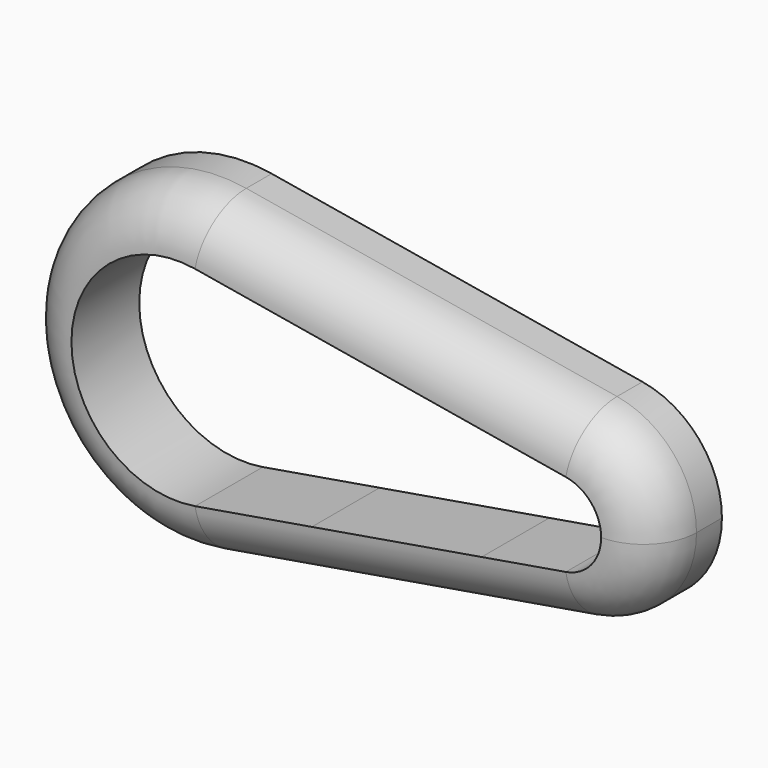
from build123d import *

# Parameters (mm, degrees)
F1_DEPTH = 8
F2_R     = 4.99999


# Not quite as in the source:
# - a fillet or chamfer is up to 0.001 mm smaller than in the source, because OpenCascade refuses the exact size


with BuildPart() as f1:
    # F0 (on Front) → F1 (new body)
    with BuildSketch(Plane.XZ):
        with BuildLine():
            ThreePointArc((-36.9956071563, -9.8601329718), (-48.6622738229, 0), (-36.9956071563, 9.8601329718))
            Line((-36.9956071563, 9.8601329718), (-25.9716433602, 7.9967429906))
            ThreePointArc((-25.9716433602, 7.9967429906), (-30.3420228558, 12.4809223955), (-36.1622738229, 14.7901994577))
            ThreePointArc((-36.1622738229, 14.7901994577), (-53.6622738229, 0), (-36.1622738229, -14.7901994577))
            ThreePointArc((-36.1622738229, -14.7901994577), (-30.3420228558, -12.4809223955), (-25.9716433602, -7.9967429906))
            Line((-25.9716433602, -7.9967429906), (-36.9956071563, -9.8601329718))
        make_face()
        with BuildLine():
            ThreePointArc((-36.1622738229, 14.7901994577), (-30.3420228558, 12.4809223955), (-25.9716433602, 7.9967429906))
            Line((-25.9716433602, 7.9967429906), (-9.9451005014, 5.2877628134))
            ThreePointArc((-9.9451005014, 5.2877628134), (-6.064590678, 8.3321209795), (-1.1622738229, 8.8741196746))
            Line((-1.1622738229, 8.8741196746), (-36.1622738229, 14.7901994577))
        make_face()
        with BuildLine():
            Line((-9.9451005014, -5.2877628134), (-25.9716433602, -7.9967429906))
            ThreePointArc((-25.9716433602, -7.9967429906), (-30.3420228558, -12.4809223955), (-36.1622738229, -14.7901994577))
            Line((-36.1622738229, -14.7901994577), (-1.1622738229, -8.8741196746))
            ThreePointArc((-1.1622738229, -8.8741196746), (-6.064590678, -8.3321209795), (-9.9451005014, -5.2877628134))
        make_face()
        with BuildLine():
            ThreePointArc((-1.1622738229, 8.8741196746), (-6.064590678, 8.3321209795), (-9.9451005014, 5.2877628134))
            Line((-9.9451005014, 5.2877628134), (-1.9956071563, 3.9440531887))
            ThreePointArc((-1.9956071563, 3.9440531887), (0.3927766404, 2.5819888975), (1.3377261771, 0))
            ThreePointArc((1.3377261771, 0), (0.3927766404, -2.5819888975), (-1.9956071563, -3.9440531887))
            Line((-1.9956071563, -3.9440531887), (-9.9451005014, -5.2877628134))
            ThreePointArc((-9.9451005014, -5.2877628134), (-6.064590678, -8.3321209795), (-1.1622738229, -8.8741196746))
            ThreePointArc((-1.1622738229, -8.8741196746), (4.2115897195, -5.8094750193), (6.3377261771, 0))
            ThreePointArc((6.3377261771, 0), (4.2115897195, 5.8094750193), (-1.1622738229, 8.8741196746))
        make_face()
    extrude(amount=F1_DEPTH)

    # F2 (radius 5 in the source; OpenCascade refuses exactly that, so slightly less here)
    f2_edges = [f1.edges().sort_by_distance(p)[0] for p in [
        (-18.662274, -8, 11.83216),
    ]]
    fillet(f2_edges, radius=F2_R)


solid = f1.part
